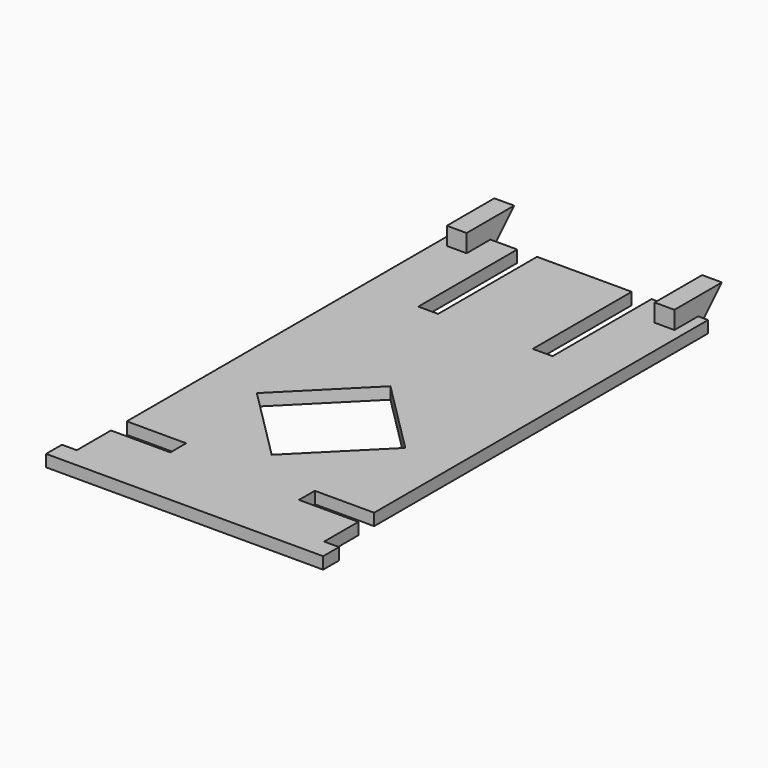
from build123d import *

# Parameters (mm, degrees)
F0_W         = 1.5
F0_H         = 2
F0_W_2       = 2
F0_H_2       = 3
F0_TEXT_SIZE = 20.8333333333
F1_DEPTH     = 1.2
F2_DEPTH     = 3
F3_SIZE      = 2.99999
F4_DEPTH     = 0.4
F5_DEPTH     = 1.2


# Not quite as in the source:
# - a fillet or chamfer is up to 0.001 mm smaller than in the source, because OpenCascade refuses the exact size
# - Text() gives the source's letters only with a copy of the font that has no kerning and outlines rounded to 1/6400 em; it was checked with that copy


with BuildPart() as f1:
    # F0 (on Top) → F1 (new body)
    with BuildSketch(Plane.XY):
        Polygon((-11.5, 25.25), (-12.5, 25.25), (-12.5, -16.9311595857), (-6.5, -16.9311595857), (-6.5, -18.9311595857), (-12.5, -18.9311595857), (-12.5, -23.25), (-12.5, -25.25), (12.5, -25.25), (12.5, -23.25), (12.5, -18.9311595857), (6.5, -18.9311595857), (6.5, -16.9311595857), (12.5, -16.9311595857), (12.5, 25.25), (11.5, 25.25), (11.5, 22.25), (9.5, 22.25), (9.5, 25.25), (6.7846251875, 25.25), (6.7846251875, 12.75), (4.7846251875, 12.75), (4.7846251875, 25.25), (-4.7846251875, 25.25), (-4.7846251875, 12.75), (-6.7846251875, 12.75), (-6.7846251875, 25.25), (-9.5, 25.25), (-9.5, 22.25), (-11.5, 22.25), align=None)
        Polygon((-7.5, -6.75), (0, 0.75), (7.5, -6.75), (0, -14.25), align=None, mode=Mode.SUBTRACT)
        Polygon((5.9163411458, 0.25), (4.1259765625, 0.25), (2.2737630208, 4.9798177083), (-3.6865234375, 4.9798177083), (-5.5159505208, 0.25), (-7.2672526042, 0.25), (-1.3883463542, 15.1848958333), (0.0667317708, 15.1848958333), align=None, mode=Mode.SUBTRACT)
        with Locations((-13.25, -24.25)):
            Rectangle(F0_W, F0_H)
        with Locations((13.25, -24.25)):
            Rectangle(F0_W, F0_H)
        with Locations((-10.5, 23.75)):
            Rectangle(F0_W_2, F0_H_2)
        with Locations((-10.5, 26.75)):
            Rectangle(F0_W_2, F0_H_2)
        with Locations((10.5, 26.75)):
            Rectangle(F0_W_2, F0_H_2)
        with Locations((10.5, 23.75)):
            Rectangle(F0_W_2, F0_H_2)
        with Locations((-7.2672526042, 0.25)):
            Text('A', F0_TEXT_SIZE, font='Open Sans', text_align=(TextAlign.LEFT, TextAlign.BOTTOM))
        with BuildLine():
            Line((-3.0745442708, 6.5358072917), (1.7366536458, 6.5358072917))
            Line((1.7366536458, 6.5358072917), (0.0048828125, 11.1451822917))
            add(Edge.make_bspline(
                [(0.0048828125, 11.1451822917), (-0.3304036458, 12.0208333333), (-0.6852213542, 13.2903645833)],
                knots=[0, 0, 0, 1, 1, 1], degree=2))
            add(Edge.make_bspline(
                [(-0.6852213542, 13.2903645833), (-0.9098307292, 12.3138020833), (-1.3264973958, 11.1451822917)],
                knots=[0, 0, 0, 1, 1, 1], degree=2))
            Line((-1.3264973958, 11.1451822917), (-3.0745442708, 6.5358072917))
        make_face()
    extrude(amount=F1_DEPTH)

    # F0 (on Top) → F2 (join)
    with BuildSketch(Plane.XY):
        with Locations((10.5, 26.75)):
            Rectangle(F0_W_2, F0_H_2)
        with Locations((-10.5, 26.75)):
            Rectangle(F0_W_2, F0_H_2)
        with Locations((10.5, 23.75)):
            Rectangle(F0_W_2, F0_H_2)
        with Locations((-10.5, 23.75)):
            Rectangle(F0_W_2, F0_H_2)
    extrude(amount=F2_DEPTH)

    # F3 (size 3 in the source; OpenCascade refuses exactly that, so slightly less here)
    f3_edges = [f1.edges().sort_by_distance(p)[0] for p in [
        (-10.5, 28.25, 0),
        (10.5, 28.25, 0),
    ]]
    chamfer(f3_edges, length=F3_SIZE)

    # F0 (on Top) → F4 (cut)
    with BuildSketch(Plane.XY):
        with Locations((-7.2672526042, 0.25)):
            Text('A', F0_TEXT_SIZE, font='Open Sans', text_align=(TextAlign.LEFT, TextAlign.BOTTOM))
    extrude(amount=F4_DEPTH, mode=Mode.SUBTRACT)

    # F0 (on Top) → F5 (join)
    with BuildSketch(Plane.XY):
        with BuildLine():
            Line((-3.0745442708, 6.5358072917), (1.7366536458, 6.5358072917))
            Line((1.7366536458, 6.5358072917), (0.0048828125, 11.1451822917))
            add(Edge.make_bspline(
                [(0.0048828125, 11.1451822917), (-0.3304036458, 12.0208333333), (-0.6852213542, 13.2903645833)],
                knots=[0, 0, 0, 1, 1, 1], degree=2))
            add(Edge.make_bspline(
                [(-0.6852213542, 13.2903645833), (-0.9098307292, 12.3138020833), (-1.3264973958, 11.1451822917)],
                knots=[0, 0, 0, 1, 1, 1], degree=2))
            Line((-1.3264973958, 11.1451822917), (-3.0745442708, 6.5358072917))
        make_face()
    extrude(amount=F5_DEPTH)


solid = f1.part
